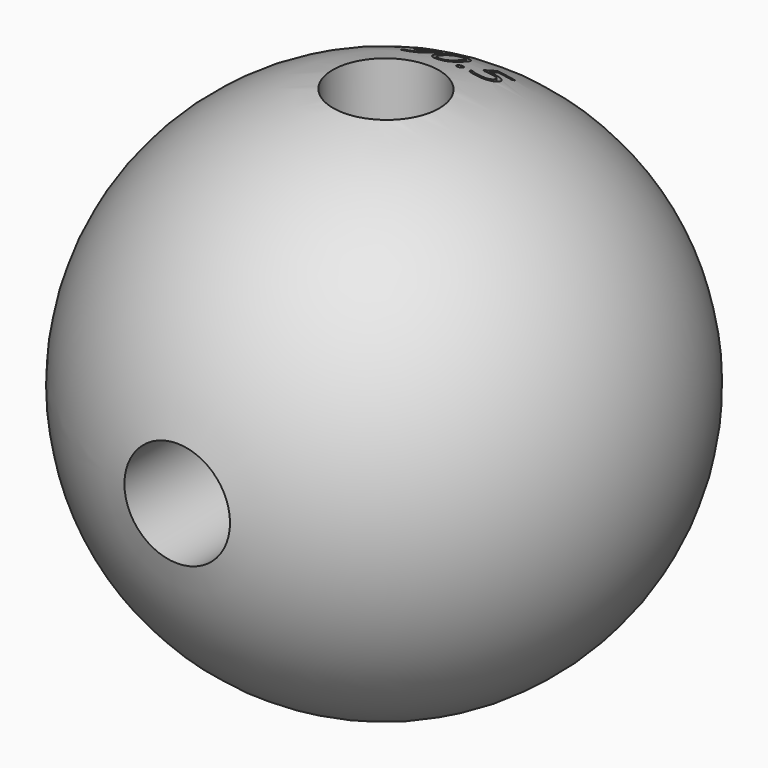
from build123d import *

# Parameters (mm, degrees)
F4_R         = 3.175
F5_DEPTH     = 25.4
F7_ANGLE     = -90.5
F9_TEXT_SIZE = 2.9445561166
F10_DEPTH    = 6.35


# Not quite as in the source:
# - Text() gives the source's letters only with a copy of the font that has no kerning and outlines rounded to 1/6400 em; it was checked with that copy


with BuildPart() as f2:
    # F1 (on Top) → F2 (revolve)
    with BuildSketch(Plane.XY):
        with BuildLine():
            Line((0, -15.875), (0, 15.875))
            ThreePointArc((0, 15.875), (-15.875, 0), (0, -15.875))
        make_face()
    revolve(axis=Axis((0, 0, 0), (0, -1, 0)))

    # F9 (on offset) → F10 (cut)
    with BuildSketch(Plane(origin=(0, 0.1662405012, 19.0492746344), x_dir=(1, 0, 0), z_dir=(0, 0.0087265355, 0.9999619231))):
        with Locations((-2.9957653023, 4.4706054032)):
            Text('90.5', F9_TEXT_SIZE, font='Open Sans', text_align=(TextAlign.LEFT, TextAlign.BOTTOM))
    extrude(amount=-F10_DEPTH, mode=Mode.SUBTRACT)


with BuildPart() as f5:
    # F4 (on offset) → F5 (new body)
    with BuildSketch(Plane.XZ.offset(6.35)):
        Circle(F4_R)
    extrude(amount=F5_DEPTH)


with BuildPart() as f7_1:
    # F7: copy of F5
    add(f5.part.rotate(Axis((28.7593565881, 0, 0), (1, 0, 0)), F7_ANGLE))


with BuildPart() as f2_1:
    add(f2.part)

    # F11: cut F7_1, F5
    add(f7_1.part, mode=Mode.SUBTRACT)
    add(f5.part, mode=Mode.SUBTRACT)


solid = f2_1.part
